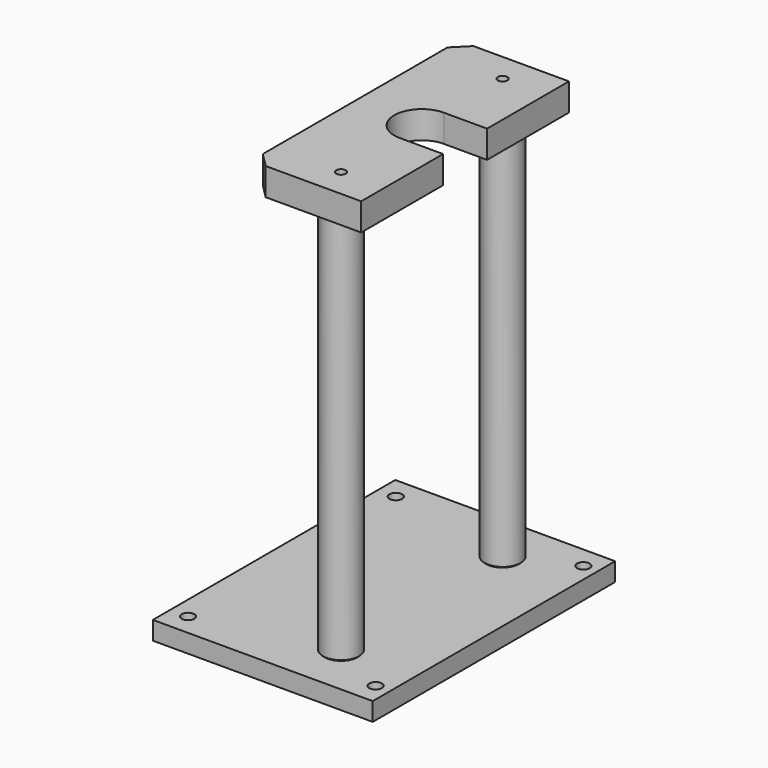
from build123d import *

# Parameters (mm, degrees)
F2_W            = 152.4
F2_H            = 210
F4_DEPTH        = 12.7
F5_R            = 12.5
F6_DEPTH        = 287.3
F7_DEPTH        = 287.3
F8_SIZE         = 1
F9_SIZE         = 1
F10_D           = 5
F10_DEPTH       = 15
F10_TIP         = 1.5021515476
F11_D           = 5
F11_DEPTH       = 15
F11_TIP         = 1.5021515476
F12_D           = 6.6
F12_DEPTH       = 15
F12_CBORE_D     = 11.25
F12_CBORE_DEPTH = 6
F12_TIP         = 1.9828400428
F14_D           = 5
F14_DEPTH       = 15
F14_TIP         = 1.5021515476
F14_2_D         = 5
F14_2_DEPTH     = 15
F14_2_TIP       = 1.5021515476
F15_DEPTH       = 14
F15_DEPTH_BACK  = 5.05
F16_R           = 12.5
F17_DEPTH       = 300.001
F19_D           = 6.6
F20_SIZE        = 10
F22_D           = 8.8


with BuildPart() as f4:
    # F2 (on Top) → F4 (new body, through all)
    with BuildSketch(Plane.XY):
        with Locations((-26.2, 0)):
            Rectangle(F2_W, F2_H)
    extrude(amount=F4_DEPTH)

    # F12
    with Locations(Plane(origin=(0, 0, 0), x_dir=(1, 0, 0), z_dir=(0, 0, -1))):
        with Locations((0, 70), (0, -70)):
            CounterBoreHole(F12_D / 2, F12_CBORE_D / 2, F12_CBORE_DEPTH, depth=F12_DEPTH)
            with Locations((0, 0, -(F12_DEPTH + F12_TIP / 2))):  # 118° drill point
                Cone(0, F12_D / 2, F12_TIP, mode=Mode.SUBTRACT)

    # F22 (through all)
    with Locations(Plane.XY.offset(12.7)):
        with Locations((-90, 90), (-90, -90), (40, -90), (40, 90)):
            Hole(F22_D / 2)


with BuildPart() as f6:
    # F5 (on offset) → F6 (new body, through all)
    with BuildSketch(Plane.XY.offset(12.7)):
        with Locations((0, 70)):
            Circle(F5_R)
    extrude(amount=F6_DEPTH)

    # F8
    f8_edges = [f6.edges().sort_by_distance(p)[0] for p in [
        (-12.5, 70, 12.7),
        (-12.5, 70, 300),
    ]]
    chamfer(f8_edges, length=F8_SIZE)

    # F10
    with Locations(Plane(origin=(0, 0, 12.7), x_dir=(1, 0, 0), z_dir=(0, 0, -1))):
        with Locations((0, -70)):
            Hole(F10_D / 2, depth=F10_DEPTH)
            with Locations((0, 0, -(F10_DEPTH + F10_TIP / 2))):  # 118° drill point
                Cone(0, F10_D / 2, F10_TIP, mode=Mode.SUBTRACT)

    # F14
    with Locations(Plane.XY.offset(300)):
        with Locations((0, -70.14721632), (0, 70)):
            Hole(F14_D / 2, depth=F14_DEPTH)
            with Locations((0, 0, -(F14_DEPTH + F14_TIP / 2))):  # 118° drill point
                Cone(0, F14_D / 2, F14_TIP, mode=Mode.SUBTRACT)


with BuildPart() as f7:
    # F5 (on offset) → F7 (new body, through all)
    with BuildSketch(Plane.XY.offset(12.7)):
        with Locations((0, -70)):
            Circle(F5_R)
    extrude(amount=F7_DEPTH)

    # F9
    f9_edges = [f7.edges().sort_by_distance(p)[0] for p in [
        (-12.5, -70, 12.7),
        (-12.5, -70, 300),
    ]]
    chamfer(f9_edges, length=F9_SIZE)

    # F11
    with Locations(Plane(origin=(0, 0, 12.7), x_dir=(1, 0, 0), z_dir=(0, 0, -1))):
        with Locations((0, 70)):
            Hole(F11_D / 2, depth=F11_DEPTH)
            with Locations((0, 0, -(F11_DEPTH + F11_TIP / 2))):  # 118° drill point
                Cone(0, F11_D / 2, F11_TIP, mode=Mode.SUBTRACT)

    # F14#2
    with Locations(Plane.XY.offset(300)):
        with Locations((0, -70.14721632), (0, 70)):
            Hole(F14_2_D / 2, depth=F14_2_DEPTH)
            with Locations((0, 0, -(F14_2_DEPTH + F14_2_TIP / 2))):  # 118° drill point
                Cone(0, F14_2_D / 2, F14_2_TIP, mode=Mode.SUBTRACT)


with BuildPart() as f15:
    # F3 (on offset) → F15 (new body, two sides)
    with BuildSketch(Plane.XY.offset(300)) as f15_sk:
        with BuildLine():
            Line((30, 19.05), (30, 90))
            Line((30, 90), (-46.2, 90))
            Line((-46.2, 90), (-46.2, -90))
            Line((-46.2, -90), (30, -90))
            Line((30, -90), (30, -19.05))
            Line((30, -19.05), (0, -19.05))
            ThreePointArc((0, -19.05), (-19.05, 0), (0, 19.05))
            Line((0, 19.05), (30, 19.05))
        make_face()
    extrude(amount=-F15_DEPTH)
    extrude(f15_sk.sketch, amount=F15_DEPTH_BACK)

    # F16 (on offset) + F15_face (on face) → F17 (cut, through all)
    with BuildSketch(Plane.XY.offset(300)):
        with Locations((0, -70)):
            Circle(F16_R)
        with Locations((0, 70)):
            Circle(F16_R)
    with BuildSketch(Plane(origin=(-10.3004424881, 0, 286), x_dir=(1, 0, 0), z_dir=(0, 0, -1))):
        with BuildLine():
            Line((40.3004424881, -90), (40.3004424881, -19.05))
            Line((40.3004424881, -19.05), (10.3004424881, -19.05))
            ThreePointArc((10.3004424881, -19.05), (-8.7495575119, 0), (10.3004424881, 19.05))
            Line((10.3004424881, 19.05), (40.3004424881, 19.05))
            Line((40.3004424881, 19.05), (40.3004424881, 90))
            Line((40.3004424881, 90), (-35.8995575119, 90))
            Line((-35.8995575119, 90), (-35.8995575119, -90))
            Line((-35.8995575119, -90), (40.3004424881, -90))
        make_face()
    extrude(amount=-F17_DEPTH, dir=(0, 0, 1), mode=Mode.SUBTRACT)

    # F19 (through all)
    with Locations(Plane.XY.offset(305.05)):
        with Locations((0, 70), (0, -70)):
            Hole(F19_D / 2)

    # F20
    f20_edges = [f15.edges().sort_by_distance(p)[0] for p in [
        (-46.2, 90, 295.525),
        (-46.2, -90, 295.525),
    ]]
    chamfer(f20_edges, length=F20_SIZE)


solid = Compound([f4.part, f6.part, f7.part, f15.part])
